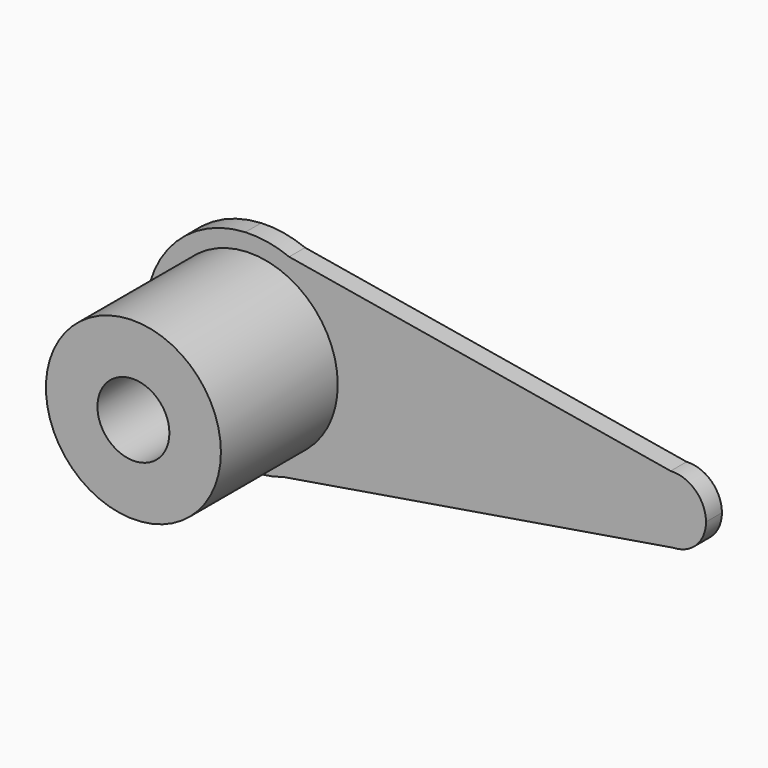
from build123d import *

# Parameters (mm, degrees)
F0_R     = 13.1802136703
F0_R_2   = 5.4198051915
F1_DEPTH = 25
F2_DEPTH = 3


# Not quite as in the source:
# - the program builds the solid bodies; features that only make, move or delete a surface that nothing else refers to are left out


with BuildPart() as f1:
    # F0 (on Front) → F1 (new body)
    with BuildSketch(Plane.XZ):
        with Locations((-42.5139516592, 0)):
            Circle(F0_R)
        with Locations((-42.5139516592, 0)):
            Circle(F0_R_2, mode=Mode.SUBTRACT)
    extrude(amount=F1_DEPTH)


with BuildPart() as f2:
    # F0 (on Front) → F2 (new body)
    with BuildSketch(Plane.XZ):
        with BuildLine():
            Line((20.8140872557, 4.8713734487), (-36.6541866123, 14.585258601))
            ThreePointArc((-36.6541866123, 14.585258601), (-29.4914236938, 8.8022940336), (-26.7955988555, 0))
            ThreePointArc((-26.7955988555, 0), (-29.7352710301, -9.1527010353), (-37.454722911, -14.8818956903))
            Line((-37.454722911, -14.8818956903), (21.2636660443, -5.1729371042))
            ThreePointArc((21.2636660443, -5.1729371042), (16.0867370449, -0.3724373523), (20.8140872557, 4.8713734487))
        make_face()
        with BuildLine():
            Line((-37.454722911, -14.8818956903), (-42.5134955187, -15.7183527971))
            ThreePointArc((-42.5134955187, -15.7183527971), (-39.9497718846, -15.5077914916), (-37.454722911, -14.8818956903))
        make_face()
        with BuildLine():
            ThreePointArc((26.1370662263, -0.1476258039), (24.5585090431, 3.5103947885), (20.8140872557, 4.8713734487))
            ThreePointArc((20.8140872557, 4.8713734487), (16.0867370449, -0.3724373523), (21.2636660443, -5.1729371042))
            ThreePointArc((21.2636660443, -5.1729371042), (24.7186267901, -3.6477609084), (26.1370662263, -0.1476258039))
        make_face()
        with BuildLine():
            ThreePointArc((-36.6541866123, 14.585258601), (-39.8942330305, 15.4985060302), (-43.2544350848, 15.7009012212))
            Line((-43.2544350848, 15.7009012212), (-36.6541866123, 14.585258601))
        make_face()
        with BuildLine():
            Line((-36.6541866123, 14.585258601), (-43.2544350848, 15.7009012212))
            ThreePointArc((-43.2544350848, 15.7009012212), (-58.2279355864, -0.3705725294), (-42.5134955187, -15.7183527971))
            Line((-42.5134955187, -15.7183527971), (-37.454722911, -14.8818956903))
            ThreePointArc((-37.454722911, -14.8818956903), (-29.7352710301, -9.1527010353), (-26.7955988555, 0))
            ThreePointArc((-26.7955988555, 0), (-29.4914236938, 8.8022940336), (-36.6541866123, 14.585258601))
        make_face()
        with Locations((-42.5139516592, 0)):
            Circle(F0_R, mode=Mode.SUBTRACT)
    extrude(amount=F2_DEPTH)


solid = Compound([f1.part, f2.part])
